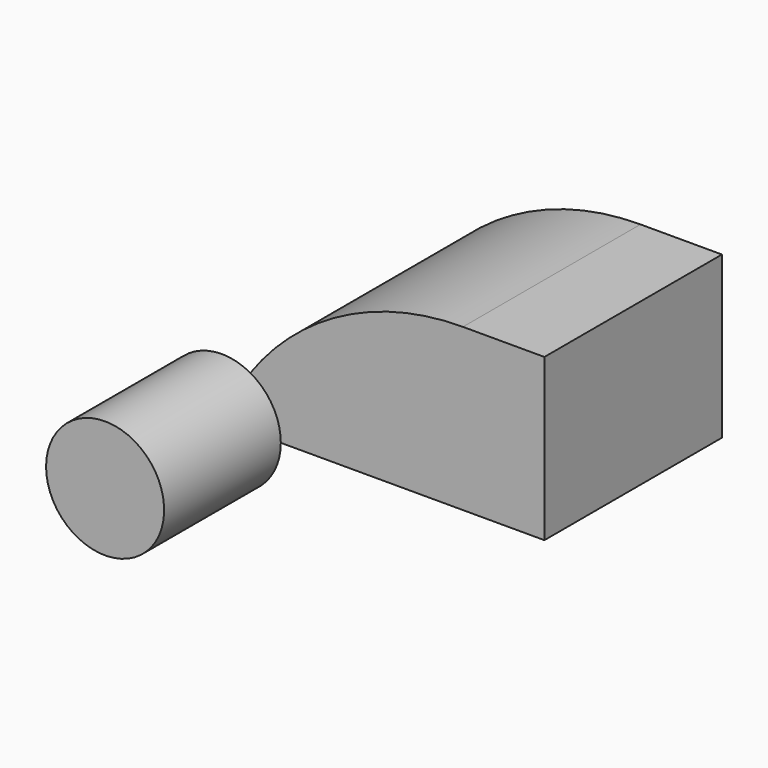
from build123d import *

# Parameters (mm, degrees)
F0_W        = 50.8
F0_H        = 34.9398194141
F1_DEPTH    = 25.4
F0_W_2      = 9.2941272077
F0_H_2      = 22.9654247603
F3_T1_DEPTH = 129.872769086


# Not quite as in the source:
# - a fillet or chamfer that OpenCascade refuses, or shapes differently, is made with other operations: its cross-section is extruded or revolved along the edge and cut away or added


with BuildPart() as f1:
    # F0 (on Top) → F1 (new body)
    with BuildSketch(Plane.XY):
        with Locations((34.6941272077, 40.4353344673)):
            Rectangle(F0_W, F0_H)
    extrude(amount=F1_DEPTH)

    # F0 (on Top) → F2 (revolve)
    with BuildSketch(Plane.XY):
        with Locations((4.6470636039, 11.4827123801)):
            Rectangle(F0_W_2, F0_H_2)
    revolve(axis=Axis((9.2941272077, 11.4827123801, 0), (0, 1, 0)))

    # F3: fillet of radius 41.0850864045 on 1 edges, made by hand

    # F3_s2 → F3_t1 (cut)
    with BuildSketch(Plane.XZ.offset(-152.8381938463)):
        with BuildLine():
            ThreePointArc((9.2941272077, 0), (24.4247897604, 18.4646387412), (47.2673070765, 25.4))
            Line((47.2673070765, 25.4), (9.2941272077, 25.4))
            Line((9.2941272077, 25.4), (9.2941272077, 0))
        make_face()
    extrude(amount=F3_T1_DEPTH, mode=Mode.SUBTRACT)


solid = f1.part
